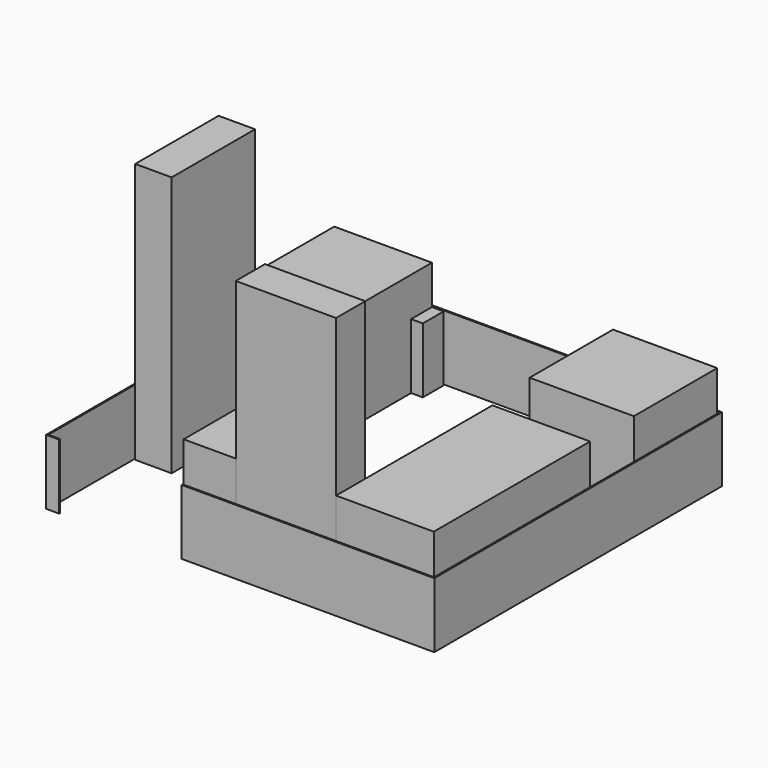
from build123d import *

# Parameters (mm, degrees)
F1_DEPTH = 500
F0_W     = 280
F0_H     = 800
F2_DEPTH = 2000
F0_W_2   = 90
F0_H_2   = 200
F3_DEPTH = 500
F0_W_3   = 670
F4_DEPTH = 800
F0_W_4   = 770
F0_H_3   = 280
F5_DEPTH = 2000
F6_DEPTH = 800
F0_W_5   = 800
F7_DEPTH = 800
F0_W_6   = 30
F8_DEPTH = 800


with BuildPart() as f1:
    # F0 (on Top) → F1 (new body)
    with BuildSketch(Plane.XY):
        Polygon((-1490, -750), (-1490, 1990), (1470, 1990), (1470, -750), (-460, -750), (-460, -760), (1480, -760), (1480, 2000), (-1500, 2000), (-1500, -760), (-1400, -760), (-1400, -750), align=None)
    extrude(amount=F1_DEPTH)


with BuildPart() as f2:
    # F0 (on Top) → F2 (new body)
    with BuildSketch(Plane.XY):
        with Locations((-1340, 470)):
            Rectangle(F0_W, F0_H)
    extrude(amount=F2_DEPTH)


with BuildPart() as f3:
    # F0 (on Top) → F3 (new body)
    with BuildSketch(Plane.XY):
        with Locations((-685, 1880)):
            Rectangle(F0_W_2, F0_H_2)
    extrude(amount=F3_DEPTH)


with BuildPart() as f4:
    # F0 (on Top) → F4 (new body)
    with BuildSketch(Plane.XY):
        with Locations((-1065, 1880)):
            Rectangle(F0_W_3, F0_H_2)
        Polygon((-1400, 1780), (-1400, 1980), (-1480, 1980), (-1480, 880), (-730, 880), (-730, 1780), align=None)
    extrude(amount=F4_DEPTH)


with BuildPart() as f5:
    # F0 (on Top) → F5 (new body)
    with BuildSketch(Plane.XY):
        with Locations((325, -600)):
            Rectangle(F0_W_4, F0_H_3)
    extrude(amount=F5_DEPTH)


with BuildPart() as f6:
    # F0 (on Top) → F6 (new body)
    with BuildSketch(Plane.XY):
        Polygon((1460, 760), (710, 760), (710, -460), (710, -740), (1460, -740), align=None)
    extrude(amount=F6_DEPTH)


with BuildPart() as f7:
    # F0 (on Top) → F7 (new body)
    with BuildSketch(Plane.XY):
        with Locations((1060, 1580)):
            Rectangle(F0_W_5, F0_H)
    extrude(amount=F7_DEPTH)


with BuildPart() as f8:
    # F0 (on Top) → F8 (new body)
    with BuildSketch(Plane.XY):
        Polygon((-90, -460), (-60, -460), (-60, -240), (-460, -240), (-460, -740), (-90, -740), align=None)
        with Locations((-75, -600)):
            Rectangle(F0_W_6, F0_H_3)
    extrude(amount=F8_DEPTH)


solid = Compound([f1.part, f2.part, f3.part, f4.part, f5.part, f6.part, f7.part, f8.part])
